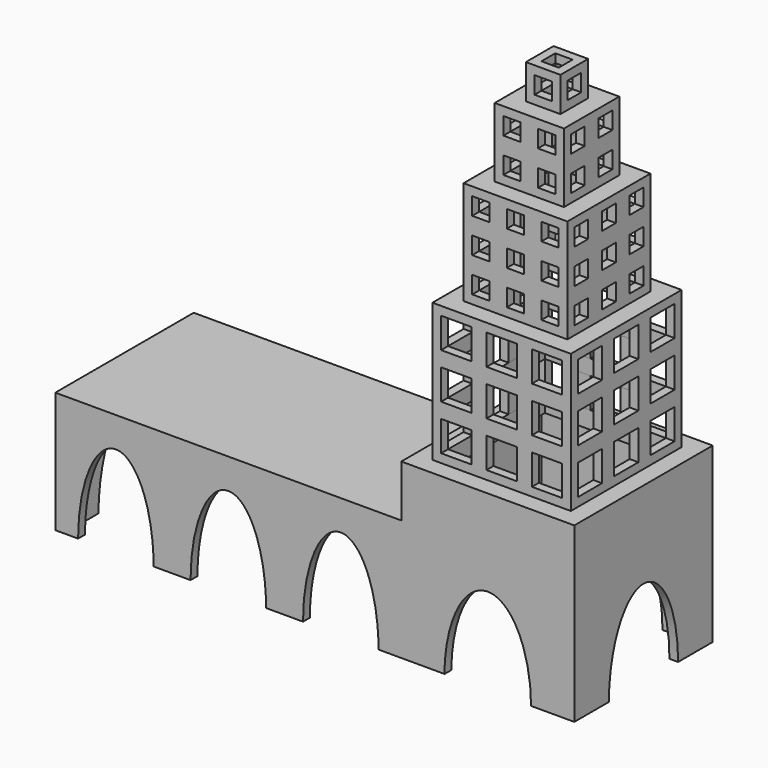
from build123d import *

# Parameters (mm, degrees)
F0_W      = 127
F0_H      = 127
F1_DEPTH  = 63.5
F2_W      = 101.6
F2_H      = 101.6
F3_DEPTH  = 101.6
F4_W      = 76.2
F4_H      = 76.2
F5_DEPTH  = 76.2
F6_W      = 50.8
F6_H      = 50.8
F7_DEPTH  = 50.8
F8_W      = 25.4
F8_H      = 25.4
F9_DEPTH  = 25.4
F10_T     = -6.35
F11_W     = 127
F11_H     = 88.9
F12_DEPTH = 254
F14_T     = -6.35
F15_DEPTH = 381.001
F17_DEPTH = 127
F18_W     = 22.225
F18_H     = 22.225
F19_DEPTH = 114.3010001
F20_W     = 22.225
F20_H     = 22.225
F21_DEPTH = 114.3010001
F22_W     = 12.7
F22_H     = 12.7
F23_DEPTH = 76.2010001
F24_W     = 12.7
F24_H     = 12.7
F25_DEPTH = 76.2010001
F27_DEPTH = 127.0010001
F28_W     = 12.7
F28_H     = 12.7
F29_DEPTH = 101.6010001
F30_W     = 12.7
F30_H     = 12.7
F31_DEPTH = 101.6010001
F32_W     = 12.7
F32_H     = 12.7
F33_DEPTH = 88.9010001
F34_W     = 12.7
F34_H     = 12.7
F35_DEPTH = 88.9010001
F36_W     = 12.7
F36_H     = 12.7
F37_DEPTH = 25.4


# Not quite as in the source:
# - a shell that OpenCascade refuses in one call is made with other operations: the cavity is built on its own and cut out


with BuildPart() as f1:
    # F0 (on Front) → F1 (new body, symmetric)
    with BuildSketch(Plane.XZ):
        Rectangle(F0_W, F0_H)
    extrude(amount=F1_DEPTH, both=True)

    # F2 (on face) → F3 (join)
    with BuildSketch(Plane.XY.offset(63.5)):
        Rectangle(F2_W, F2_H)
    extrude(amount=F3_DEPTH)

    # F4 (on face) → F5 (join)
    with BuildSketch(Plane.XY.offset(165.1)):
        Rectangle(F4_W, F4_H)
    extrude(amount=F5_DEPTH)

    # F6 (on face) → F7 (join)
    with BuildSketch(Plane.XY.offset(241.3)):
        Rectangle(F6_W, F6_H)
    extrude(amount=F7_DEPTH)

    # F8 (on face) → F9 (join)
    with BuildSketch(Plane.XY.offset(292.1)):
        Rectangle(F8_W, F8_H)
    extrude(amount=F9_DEPTH)

    # F10
    f10_openings = [f1.faces().sort_by_distance(p)[0] for p in [
        (0, 0, -63.5),
    ]]
    offset(amount=F10_T, openings=f10_openings, kind=Kind.INTERSECTION)

    # F11 (on face) → F12 (join)
    with BuildSketch(Plane(origin=(-63.5, 0, 0), x_dir=(0, -1, 0), z_dir=(-1, 0, 0))):
        with Locations((0, -19.05)):
            Rectangle(F11_W, F11_H)
    extrude(amount=F12_DEPTH)

    # F14: a shell. OpenCascade refuses it in one call, so the cavity is built on its own and cut out:
    # the body offset inwards by the wall thickness, plus a prism from it out through each open face.
    f14_core = offset(f1.part, amount=F14_T, kind=Kind.INTERSECTION, mode=Mode.PRIVATE)
    f14_exits = [f14_core.faces().sort_by_distance(p)[0] for p in [
        (-187.325, 0, -57.15),
    ]]
    add(f14_core, mode=Mode.SUBTRACT)
    extrude(f14_exits, amount=-F14_T, mode=Mode.SUBTRACT)

    # F13 (on face) → F15 (cut, through all)
    with BuildSketch(Plane(origin=(-317.5, 0, 0), x_dir=(0, -1, 0), z_dir=(-1, 0, 0))):
        with BuildLine():
            add(Edge.make_bspline(
                [(0, 0), (-54.9926131403, 0), (-27.4963065702, -95.25), (0, -190.5), (27.4963065702, -95.25), (54.9926131403, 0), (0, 0)],
                knots=[0, 0, 0, 2.0943951024, 2.0943951024, 4.1887902048, 4.1887902048, 6.2831853072, 6.2831853072, 6.2831853072], degree=2, weights=[1, 0.5, 1, 0.5, 1, 0.5, 1]))
        make_face()
    extrude(amount=-F15_DEPTH, mode=Mode.SUBTRACT)

    # F16 (on face) → F17 (cut)
    with BuildSketch(Plane(origin=(0, 63.5, 0), x_dir=(-1, 0, 0), z_dir=(0, 1, 0))):
        with BuildLine():
            add(Edge.make_bspline(
                [(218.2221051752, -63.5), (218.2221051752, 3.175), (190.5, 3.175), (162.7778948248, 3.175), (162.7778948248, -63.5)],
                knots=[4.7123889804, 4.7123889804, 4.7123889804, 6.2831853072, 6.2831853072, 7.853981634, 7.853981634, 7.853981634], degree=2, weights=[1, 0.7071067812, 1, 0.7071067812, 1]))
            Line((162.7778948248, -63.5), (218.2221051752, -63.5))
        make_face()
        with BuildLine():
            Line((245.3278948248, -63.5), (300.7721051752, -63.5))
            add(Edge.make_bspline(
                [(300.7721051752, -63.5), (300.7721051752, 3.175), (273.05, 3.175), (245.3278948248, 3.175), (245.3278948248, -63.5)],
                knots=[4.7123889804, 4.7123889804, 4.7123889804, 6.2831853072, 6.2831853072, 7.853981634, 7.853981634, 7.853981634], degree=2, weights=[1, 0.7071067812, 1, 0.7071067812, 1]))
        make_face()
        with BuildLine():
            Line((80.2278948248, -63.5), (135.6721051752, -63.5))
            add(Edge.make_bspline(
                [(135.6721051752, -63.5), (135.6721051752, 3.175), (107.95, 3.175), (80.2278948248, 3.175), (80.2278948248, -63.5)],
                knots=[4.7123889804, 4.7123889804, 4.7123889804, 6.2831853072, 6.2831853072, 7.853981634, 7.853981634, 7.853981634], degree=2, weights=[1, 0.7071067812, 1, 0.7071067812, 1]))
        make_face()
    extrude(amount=-F17_DEPTH, mode=Mode.SUBTRACT)

    # F18 (on face) → F19 (cut, through all)
    with BuildSketch(Plane(origin=(0, 50.8, 0), x_dir=(-1, 0, 0), z_dir=(0, 1, 0))):
        with Locations((-33.3375, 147.6375)):
            Rectangle(F18_W, F18_H)
        with Locations((0, 147.6375)):
            Rectangle(F18_W, F18_H)
        with Locations((33.3375, 147.6375)):
            Rectangle(F18_W, F18_H)
        with Locations((33.3375, 114.3)):
            Rectangle(F18_W, F18_H)
        with Locations((0, 114.3)):
            Rectangle(F18_W, F18_H)
        with Locations((-33.3375, 114.3)):
            Rectangle(F18_W, F18_H)
        with Locations((-33.3375, 80.9625)):
            Rectangle(F18_W, F18_H)
        with Locations((0, 80.9625)):
            Rectangle(F18_W, F18_H)
        with Locations((33.3375, 80.9625)):
            Rectangle(F18_W, F18_H)
    extrude(amount=-F19_DEPTH, mode=Mode.SUBTRACT)

    # F20 (on face) → F21 (cut, through all)
    with BuildSketch(Plane(origin=(-50.8, 0, 0), x_dir=(0, -1, 0), z_dir=(-1, 0, 0))):
        with Locations((-33.3375, 147.6375)):
            Rectangle(F20_W, F20_H)
        with Locations((0, 147.6375)):
            Rectangle(F20_W, F20_H)
        with Locations((33.3375, 147.6375)):
            Rectangle(F20_W, F20_H)
        with Locations((-33.3375, 114.3)):
            Rectangle(F20_W, F20_H)
        with Locations((0, 114.3)):
            Rectangle(F20_W, F20_H)
        with Locations((33.3375, 114.3)):
            Rectangle(F20_W, F20_H)
        with Locations((-33.3375, 80.9625)):
            Rectangle(F20_W, F20_H)
        with Locations((0, 80.9625)):
            Rectangle(F20_W, F20_H)
        with Locations((33.3375, 80.9625)):
            Rectangle(F20_W, F20_H)
    extrude(amount=-F21_DEPTH, mode=Mode.SUBTRACT)

    # F22 (on face) → F23 (cut, through all)
    with BuildSketch(Plane(origin=(0, 12.7, 0), x_dir=(-1, 0, 0), z_dir=(0, 1, 0))):
        with Locations((0, 304.8)):
            Rectangle(F22_W, F22_H)
    extrude(amount=-F23_DEPTH, mode=Mode.SUBTRACT)

    # F24 (on face) → F25 (cut, through all)
    with BuildSketch(Plane(origin=(-12.7, 0, 0), x_dir=(0, -1, 0), z_dir=(-1, 0, 0))):
        with Locations((0, 304.8)):
            Rectangle(F24_W, F24_H)
    extrude(amount=-F25_DEPTH, mode=Mode.SUBTRACT)

    # F26 (on face) → F27 (cut, through all)
    with BuildSketch(Plane(origin=(0, 63.5, 0), x_dir=(-1, 0, 0), z_dir=(0, 1, 0))):
        with BuildLine():
            add(Edge.make_bspline(
                [(0, 0), (-54.9926131403, 0), (-27.4963065702, -95.25), (0, -190.5), (27.4963065702, -95.25), (54.9926131403, 0), (0, 0)],
                knots=[0, 0, 0, 2.0943951024, 2.0943951024, 4.1887902048, 4.1887902048, 6.2831853072, 6.2831853072, 6.2831853072], degree=2, weights=[1, 0.5, 1, 0.5, 1, 0.5, 1]))
        make_face()
    extrude(amount=-F27_DEPTH, mode=Mode.SUBTRACT)

    # F28 (on face) → F29 (cut, through all)
    with BuildSketch(Plane(origin=(0, 38.1, 0), x_dir=(-1, 0, 0), z_dir=(0, 1, 0))):
        with Locations((-25.4, 228.6)):
            Rectangle(F28_W, F28_H)
        with Locations((-25.4, 203.2)):
            Rectangle(F28_W, F28_H)
        with Locations((-25.4, 177.8)):
            Rectangle(F28_W, F28_H)
        with Locations((0, 177.8)):
            Rectangle(F28_W, F28_H)
        with Locations((0, 203.2)):
            Rectangle(F28_W, F28_H)
        with Locations((0, 228.6)):
            Rectangle(F28_W, F28_H)
        with Locations((25.4, 228.6)):
            Rectangle(F28_W, F28_H)
        with Locations((25.4, 203.2)):
            Rectangle(F28_W, F28_H)
        with Locations((25.4, 177.8)):
            Rectangle(F28_W, F28_H)
    extrude(amount=-F29_DEPTH, mode=Mode.SUBTRACT)

    # F30 (on face) → F31 (cut, through all)
    with BuildSketch(Plane(origin=(-38.1, 0, 0), x_dir=(0, -1, 0), z_dir=(-1, 0, 0))):
        with Locations((-25.4, 228.6)):
            Rectangle(F30_W, F30_H)
        with Locations((0, 228.6)):
            Rectangle(F30_W, F30_H)
        with Locations((25.4, 228.6)):
            Rectangle(F30_W, F30_H)
        with Locations((25.4, 203.2)):
            Rectangle(F30_W, F30_H)
        with Locations((0, 203.2)):
            Rectangle(F30_W, F30_H)
        with Locations((0, 177.8)):
            Rectangle(F30_W, F30_H)
        with Locations((-25.4, 177.8)):
            Rectangle(F30_W, F30_H)
        with Locations((-25.4, 203.2)):
            Rectangle(F30_W, F30_H)
        with Locations((25.4, 177.8)):
            Rectangle(F30_W, F30_H)
    extrude(amount=-F31_DEPTH, mode=Mode.SUBTRACT)

    # F32 (on face) → F33 (cut, through all)
    with BuildSketch(Plane(origin=(0, 25.4, 0), x_dir=(-1, 0, 0), z_dir=(0, 1, 0))):
        with Locations((-12.7, 279.4)):
            Rectangle(F32_W, F32_H)
        with Locations((-12.7, 254)):
            Rectangle(F32_W, F32_H)
        with Locations((12.7, 254)):
            Rectangle(F32_W, F32_H)
        with Locations((12.7, 279.4)):
            Rectangle(F32_W, F32_H)
    extrude(amount=-F33_DEPTH, mode=Mode.SUBTRACT)

    # F34 (on face) → F35 (cut, through all)
    with BuildSketch(Plane(origin=(-25.4, 0, 0), x_dir=(0, -1, 0), z_dir=(-1, 0, 0))):
        with Locations((-12.7, 279.4)):
            Rectangle(F34_W, F34_H)
        with Locations((-12.7, 254)):
            Rectangle(F34_W, F34_H)
        with Locations((12.7, 254)):
            Rectangle(F34_W, F34_H)
        with Locations((12.7, 279.4)):
            Rectangle(F34_W, F34_H)
    extrude(amount=-F35_DEPTH, mode=Mode.SUBTRACT)

    # F36 (on face) → F37 (cut)
    with BuildSketch(Plane.XY.offset(317.5)):
        Rectangle(F36_W, F36_H)
    extrude(amount=-F37_DEPTH, mode=Mode.SUBTRACT)


solid = f1.part
